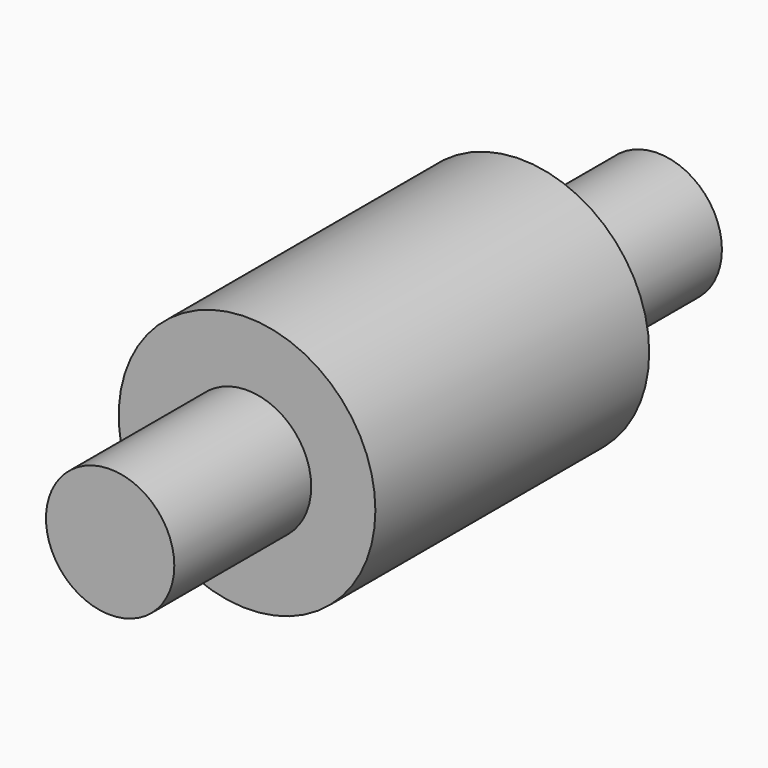
from build123d import *

# Parameters (mm, degrees)
F0_R     = 38.1
F0_R_2   = 19.05
F1_DEPTH = 50.8
F2_R     = 19.05
F3_DEPTH = 101.6


# Not quite as in the source:
# - a feature names something its author has since deleted; it is built from what else it names


with BuildPart() as f1:
    # F0 (on Front) → F1 (new body, symmetric)
    with BuildSketch(Plane.XZ):
        Circle(F0_R)
        Circle(F0_R_2, mode=Mode.SUBTRACT)
    extrude(amount=F1_DEPTH, both=True)


with BuildPart() as f3:
    # F2 (on face) → F3 (new body, symmetric)
    with BuildSketch(Plane.XZ):
        Circle(F2_R)
    extrude(amount=F3_DEPTH, both=True)


solid = Compound([f1.part, f3.part])
